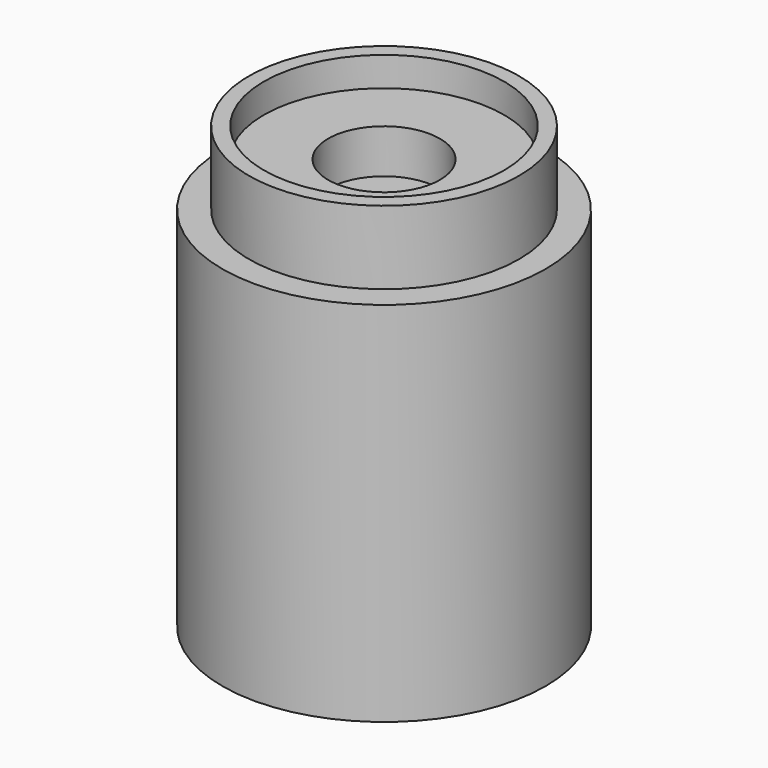
from build123d import *

# Parameters (mm, degrees)
F0_R     = 27.9540439908
F1_DEPTH = 63.5
F2_R     = 23.3610455133
F3_DEPTH = 12.7
F4_R     = 20.7815529946
F5_DEPTH = 5.08
F6_R     = 9.6661345216
F7_DEPTH = 12.7


with BuildPart() as f1:
    # F0 (on Top) → F1 (new body)
    with BuildSketch(Plane.XY):
        Circle(F0_R)
    extrude(amount=F1_DEPTH)


with BuildPart() as f3:
    # F2 (on face) → F3 (new body)
    with BuildSketch(Plane.XY.offset(63.5)):
        Circle(F2_R)
    extrude(amount=F3_DEPTH)

    # F4 (on face) → F5 (cut)
    with BuildSketch(Plane.XY.offset(76.2)):
        Circle(F4_R)
    extrude(amount=-F5_DEPTH, mode=Mode.SUBTRACT)

    # F6 (on face) → F7 (cut)
    with BuildSketch(Plane.XY.offset(71.12)):
        Circle(F6_R)
    extrude(amount=-F7_DEPTH, mode=Mode.SUBTRACT)


solid = Compound([f1.part, f3.part])
